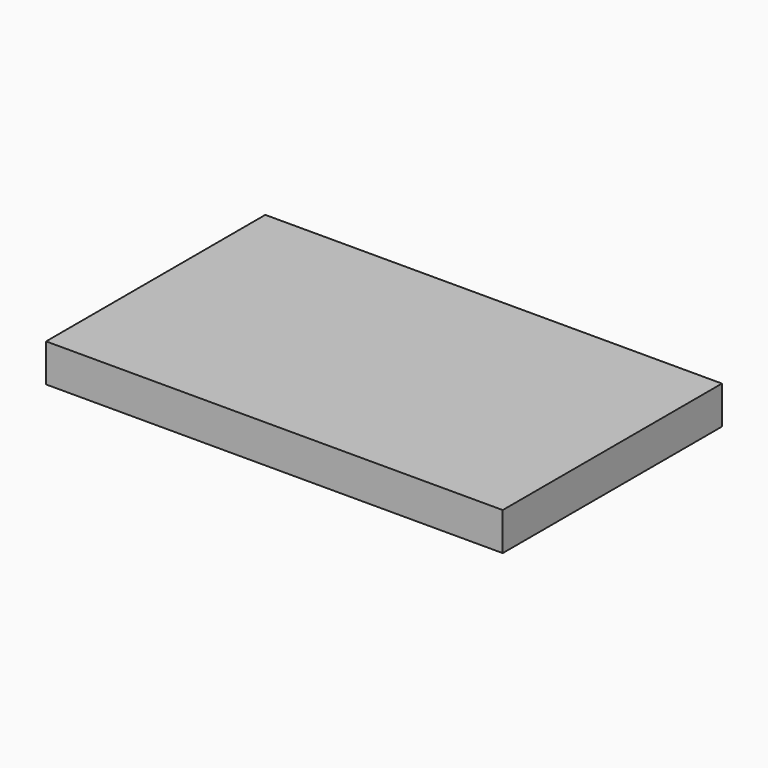
from build123d import *

# Parameters (mm, degrees)
F0_W     = 5000
F0_H     = 415.31832783
F1_DEPTH = 3000


# Not quite as in the source:
# - the program builds the solid bodies; features that only make, move or delete a surface that nothing else refers to are left out


with BuildPart() as f1:
    # F0 (on Front) → F1 (new body)
    with BuildSketch(Plane.XZ):
        Rectangle(F0_W, F0_H)
    extrude(amount=F1_DEPTH)


solid = f1.part
